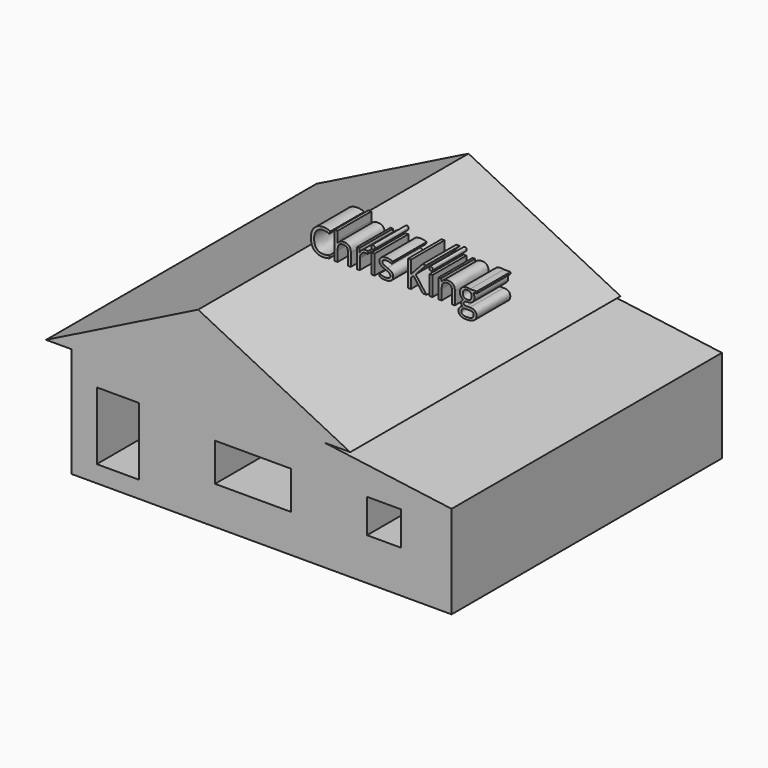
from build123d import *

# Parameters (mm, degrees)
F2_DEPTH       = 6096
F2_DEPTH_BACK  = 6096
F3_DEPTH       = 6096
F3_DEPTH_BACK  = 6096
F0_W           = 2743.2
F0_H           = 1371.6
F4_DEPTH       = 30.48
F5_DEPTH       = 6096
F5_DEPTH_BACK  = 6096
F6_DEPTH       = 609.6
F6_DEPTH_BACK  = 6096
F0_W_2         = 914.4
F0_H_2         = 2133.6
F7_DEPTH       = 609.6
F7_DEPTH_BACK  = 6217.92
F0_W_3         = 1219.2
F0_H_3         = 1219.2
F0_W_4         = 4572
F0_H_4         = 609.6
F8_DEPTH       = 6096
F8_DEPTH_BACK  = 6096
F1_W           = 914.4
F1_H           = 914.4
F9_DEPTH       = 609.6
F9_DEPTH_BACK  = 4724.4
F1_W_2         = 2438.4
F1_H_2         = 979.3705493212
F10_DEPTH      = 609.6
F10_DEPTH_BACK = 4724.4
F0_TEXT_SIZE   = 1304.4695059458
F11_DEPTH      = 1524


# Not quite as in the source:
# - Text() gives the source's letters only with a copy of the font that has no kerning and outlines rounded to 1/6400 em; it was checked with that copy


with BuildPart() as f2:
    # F0 (on Front) → F2 (new body, two sides)
    with BuildSketch(Plane.XZ) as f2_sk:
        Polygon((-5486.4, 0), (-4572, 0), (0, 2286), (0, 2743.2), align=None)
        Polygon((0, 2286), (4572, 0), (5486.4, 0), (0, 2743.2), align=None)
    extrude(amount=F2_DEPTH)
    extrude(f2_sk.sketch, amount=-F2_DEPTH_BACK)

    # F0 (on Front) → F3 (join, two sides)
    with BuildSketch(Plane.XZ) as f3_sk:
        Polygon((0, 2286), (0, 0), (4572, 0), align=None)
        Polygon((-4572, 0), (0, 0), (0, 2286), align=None)
    extrude(amount=F3_DEPTH)
    extrude(f3_sk.sketch, amount=-F3_DEPTH_BACK)

    # F0 (on Front) → F4 (join)
    with BuildSketch(Plane.XZ):
        Polygon((4572, 0), (0, 0), (-4572, 0), (-4572, -3352.8), (-3657.6, -3352.8), (-3657.6, -914.4), (-2133.6, -914.4), (-2133.6, -3352.8), (4572, -3352.8), (4572, -609.6), align=None)
        with Locations((1981.2, -1905)):
            Rectangle(F0_W, F0_H, mode=Mode.SUBTRACT)
    extrude(amount=F4_DEPTH)

    # F0 (on Front) → F5 (join, two sides)
    with BuildSketch(Plane.XZ) as f5_sk:
        Polygon((4572, 0), (0, 0), (-4572, 0), (-4572, -3352.8), (-3657.6, -3352.8), (-3657.6, -914.4), (-2133.6, -914.4), (-2133.6, -3352.8), (4572, -3352.8), (4572, -609.6), align=None)
        with Locations((1981.2, -1905)):
            Rectangle(F0_W, F0_H, mode=Mode.SUBTRACT)
        Polygon((-3657.6, -3352.8), (-4572, -3352.8), (-4572, -3962.4), (4572, -3962.4), (4572, -3352.8), (-2133.6, -3352.8), (-2438.4, -3352.8), (-3352.8, -3352.8), align=None)
    extrude(amount=F5_DEPTH)
    extrude(f5_sk.sketch, amount=-F5_DEPTH_BACK)

    # F0 (on Front) → F6 (join, two sides)
    with BuildSketch(Plane.XZ) as f6_sk:
        Polygon((-3657.6, -914.4), (-3657.6, -3352.8), (-3352.8, -3352.8), (-3352.8, -1219.2), (-2438.4, -1219.2), (-2438.4, -3352.8), (-2133.6, -3352.8), (-2133.6, -914.4), align=None)
    extrude(amount=F6_DEPTH)
    extrude(f6_sk.sketch, amount=-F6_DEPTH_BACK)

    # F0 (on Front) → F7 (join, two sides)
    with BuildSketch(Plane.XZ) as f7_sk:
        with Locations((-2895.6, -2286)):
            Rectangle(F0_W_2, F0_H_2)
    extrude(amount=F7_DEPTH)
    extrude(f7_sk.sketch, amount=-F7_DEPTH_BACK)

    # F0 (on Front) → F8 (join, two sides)
    with BuildSketch(Plane.XZ) as f8_sk:
        Polygon((9144, -1219.2), (4572, -609.6), (4572, -3352.8), (9144, -3352.8), align=None)
        with Locations((6705.6, -1828.8)):
            Rectangle(F0_W_3, F0_H_3, mode=Mode.SUBTRACT)
        Polygon((9144, -609.6), (4572, 0), (4572, -609.6), (9144, -1219.2), align=None)
        with Locations((6858, -3657.6)):
            Rectangle(F0_W_4, F0_H_4)
    extrude(amount=F8_DEPTH)
    extrude(f8_sk.sketch, amount=-F8_DEPTH_BACK)

    # F1 (on Right) → F9 (join, two sides)
    with BuildSketch(Plane.YZ) as f9_sk:
        with Locations((1289.7853162766, -708.2588915408)):
            Rectangle(F1_W, F1_H)
    extrude(amount=F9_DEPTH)
    extrude(f9_sk.sketch, amount=-F9_DEPTH_BACK)

    # F1 (on Right) → F10 (join, two sides)
    with BuildSketch(Plane.YZ) as f10_sk:
        with Locations((-2330.9179393768, -689.0083774924)):
            Rectangle(F1_W_2, F1_H_2)
    extrude(amount=F10_DEPTH)
    extrude(f10_sk.sketch, amount=-F10_DEPTH_BACK)

    # F0 (on Front) → F11 (join)
    with BuildSketch(Plane.XZ):
        Polygon((4572, 0), (0, 0), (-4572, 0), (-4572, -3352.8), (-3657.6, -3352.8), (-3657.6, -914.4), (-2133.6, -914.4), (-2133.6, -3352.8), (4572, -3352.8), (4572, -609.6), align=None)
        with Locations((1981.2, -1905)):
            Rectangle(F0_W, F0_H, mode=Mode.SUBTRACT)
        Polygon((0, 2286), (0, 0), (4572, 0), align=None)
        Polygon((-4572, 0), (0, 0), (0, 2286), align=None)
        Polygon((-5486.4, 0), (-4572, 0), (0, 2286), (0, 2743.2), align=None)
        Polygon((0, 2286), (4572, 0), (5486.4, 0), (0, 2743.2), align=None)
        Polygon((9144, -609.6), (4572, 0), (4572, -609.6), (9144, -1219.2), align=None)
        Polygon((-3657.6, -3352.8), (-4572, -3352.8), (-4572, -3962.4), (4572, -3962.4), (4572, -3352.8), (-2133.6, -3352.8), (-2438.4, -3352.8), (-3352.8, -3352.8), align=None)
        Polygon((9144, -1219.2), (4572, -609.6), (4572, -3352.8), (9144, -3352.8), align=None)
        with Locations((6705.6, -1828.8)):
            Rectangle(F0_W_3, F0_H_3, mode=Mode.SUBTRACT)
        with Locations((6858, -3657.6)):
            Rectangle(F0_W_4, F0_H_4)
        with Locations((331.8234682083, 2843.4433937073)):
            Text('Chris King', F0_TEXT_SIZE, font='Open Sans', text_align=(TextAlign.LEFT, TextAlign.BOTTOM))
    extrude(amount=F11_DEPTH)


solid = f2.part
